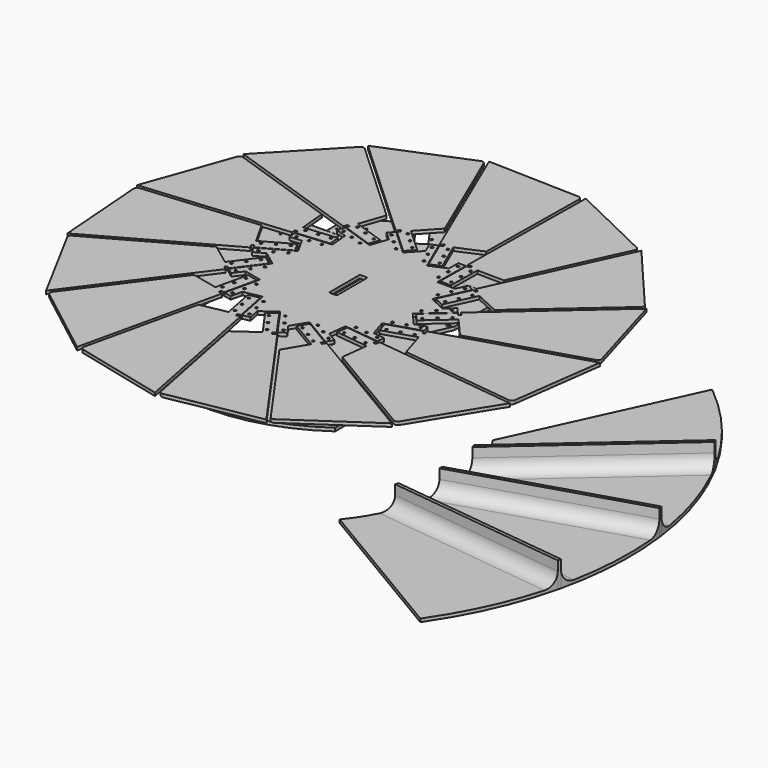
from build123d import *

# Parameters (mm, degrees)
F5_DEPTH = 40
F6_DEPTH = 35
F7_R     = 20
F0_R     = 1.9
F0_R_2   = 1.75
F8_DEPTH = 5
F2_R     = 1.4
F9_DEPTH = 5
F2_R_2   = 1.9
F2_W     = 5
F2_H     = 5
F2_R_3   = 16


with BuildPart() as f5:
    # F4 (on offset) → F5 (new body)
    with BuildSketch(Plane.XY.offset(-180)):
        with BuildLine():
            ThreePointArc((152.4859565585, -92.1641828619), (151.5670252148, -94.5763902457), (150.6219048273, -96.9784574241))
            Line((150.6219048273, -96.9784574241), (430.9555621315, -130.1581322678))
            ThreePointArc((430.9555621315, -130.1581322678), (431.541953989, -127.7107963244), (432.1163824358, -125.2606247814))
            Line((432.1163824358, -125.2606247814), (152.4859565585, -92.1641828619))
        make_face()
        with BuildLine():
            Line((430.9555621315, -130.1581322678), (150.6219048273, -96.9784574241))
            ThreePointArc((150.6219048273, -96.9784574241), (134.6384036274, -129.5048123953), (113.8875354762, -159.217394735))
            Line((113.8875354762, -159.217394735), (354.182792578, -302.1780498209))
            Line((354.182792578, -302.1780498209), (356.7392580084, -297.8810177633))
            ThreePointArc((356.7392580084, -297.8810177634), (401.3722979363, -217.3492897694), (430.9555621315, -130.1581322678))
        make_face()
        with BuildLine():
            ThreePointArc((166.581347197, -30.5797229561), (161.5926160767, -61.8432066107), (152.4859565585, -92.1641828619))
            Line((152.4859565585, -92.1641828619), (432.1163824358, -125.2606247814))
            ThreePointArc((432.1163824358, -125.2606247814), (444.73424073, -35.6541636121), (441.4771291123, 54.7776861707))
            Line((441.4771291123, 54.7776861707), (166.581347197, -30.5797229561))
        make_face()
        with BuildLine():
            ThreePointArc((167.0124499283, -25.2103692451), (166.8121368082, -27.8962695717), (166.581347197, -30.5797229561))
            Line((166.581347197, -30.5797229561), (441.4771291123, 54.7776861707))
            ThreePointArc((441.4771291123, 54.7776861707), (441.1572058027, 57.2949723658), (440.8248859522, 59.8106520411))
            Line((440.8248859522, 59.8106520411), (167.0124499283, -25.2103692451))
        make_face()
        with BuildLine():
            ThreePointArc((162.8378639859, 38.2580484491), (167.0616347314, 6.6643647704), (167.0124499283, -25.2103692451))
            Line((167.0124499283, -25.2103692451), (440.8248859522, 59.8106520411))
            ThreePointArc((440.8248859522, 59.8106520411), (420.64572605, 148.9482124367), (385.0315824556, 233.1167097719))
            Line((385.0315824556, 233.1167097719), (162.8378639859, 38.2580484491))
        make_face()
        with BuildLine():
            ThreePointArc((161.6328579843, 43.8516393894), (162.2522237752, 41.0584766059), (162.8378639859, 38.2580484491))
            Line((162.8378639859, 38.2580484491), (385.0315824556, 233.1167097719))
            ThreePointArc((385.0315824556, 233.1167097719), (383.8207285252, 235.3780934105), (382.598628532, 237.6334192868))
            Line((382.598628532, 237.6334192868), (161.6328579843, 43.8516393894))
        make_face()
        with BuildLine():
            ThreePointArc((129.2130710056, 120.4418545445), (148.8051032395, 83.578368714), (161.6328579843, 43.8516393894))
            Line((161.6328579843, 43.8516393894), (382.598628532, 237.6334192868))
            ThreePointArc((382.598628532, 237.6334192868), (327.625776734, 318.9452816199), (258.2280754908, 388.3541603965))
            Line((258.2280754908, 388.3541603965), (254.2399532921, 391.6461274173))
            Line((254.2399532921, 391.6461274173), (129.2130710056, 120.4418545445))
        make_face()
    extrude(amount=-F5_DEPTH)

    # F4 (on offset) → F6 (cut)
    with BuildSketch(Plane.XY.offset(-180)):
        with BuildLine():
            Line((430.9555621315, -130.1581322678), (150.6219048273, -96.9784574241))
            ThreePointArc((150.6219048273, -96.9784574241), (134.6384036274, -129.5048123953), (113.8875354762, -159.217394735))
            Line((113.8875354762, -159.217394735), (354.182792578, -302.1780498209))
            Line((354.182792578, -302.1780498209), (356.7392580084, -297.8810177633))
            ThreePointArc((356.7392580084, -297.8810177634), (401.3722979363, -217.3492897694), (430.9555621315, -130.1581322678))
        make_face()
        with BuildLine():
            ThreePointArc((166.581347197, -30.5797229561), (161.5926160767, -61.8432066107), (152.4859565585, -92.1641828619))
            Line((152.4859565585, -92.1641828619), (432.1163824358, -125.2606247814))
            ThreePointArc((432.1163824358, -125.2606247814), (444.73424073, -35.6541636121), (441.4771291123, 54.7776861707))
            Line((441.4771291123, 54.7776861707), (166.581347197, -30.5797229561))
        make_face()
        with BuildLine():
            ThreePointArc((162.8378639859, 38.2580484491), (167.0616347314, 6.6643647704), (167.0124499283, -25.2103692451))
            Line((167.0124499283, -25.2103692451), (440.8248859522, 59.8106520411))
            ThreePointArc((440.8248859522, 59.8106520411), (420.64572605, 148.9482124367), (385.0315824556, 233.1167097719))
            Line((385.0315824556, 233.1167097719), (162.8378639859, 38.2580484491))
        make_face()
        with BuildLine():
            ThreePointArc((129.2130710056, 120.4418545445), (148.8051032395, 83.578368714), (161.6328579843, 43.8516393894))
            Line((161.6328579843, 43.8516393894), (382.598628532, 237.6334192868))
            ThreePointArc((382.598628532, 237.6334192868), (327.625776734, 318.9452816199), (258.2280754908, 388.3541603965))
            Line((258.2280754908, 388.3541603965), (254.2399532921, 391.6461274173))
            Line((254.2399532921, 391.6461274173), (129.2130710056, 120.4418545445))
        make_face()
    extrude(amount=-F6_DEPTH, mode=Mode.SUBTRACT)

    # F7
    f7_edges = [f5.edges().sort_by_distance(p)[0] for p in [
        (290.788733, -113.568295, -215),
        (304.029238, 12.098982, -215),
        (273.934723, 135.687379, -215),
        (292.301169, -108.712404, -215),
        (303.918668, 17.300141, -215),
        (272.115743, 140.742529, -215),
    ]]
    fillet(f7_edges, radius=F7_R)


with BuildPart() as f8:
    # F0 (on Top) → F8 (new body)
    with BuildSketch(Plane.XY):
        with BuildLine():
            Line((-99.5654662237, 123.5643549186), (-95.7777457057, 122.2785970574))
            Line((-95.7777457057, 122.2785970574), (-91.9847600151, 133.4523725854))
            Line((-91.9847600151, 133.4523725854), (-78.5983493232, 172.8874668356))
            Line((-78.5983493232, 172.8874668356), (-209.6199457093, 294.0025847368))
            ThreePointArc((-209.6199457093, 294.0025847368), (-213.166642003, 295.3286401438), (-216.6257692473, 293.7885374685))
            Line((-216.6257692473, 293.7885374685), (-315.5944341041, 190.1376257037))
            Line((-315.5944341041, 190.1376257037), (-101.6226788016, 117.5040020898))
            Line((-101.6226788016, 117.5040020898), (-99.5654662237, 123.5643549186))
        make_face()
        Polygon((-96.099185171, 121.3316669279), (-97.5135188184, 117.1651743581), (-49.2200822141, 100.7717616276), (-47.8057485668, 104.9382541974), align=None)
        Polygon((-95.7777457057, 122.2785970574), (-96.099185171, 121.3316669279), (-47.8057485668, 104.9382541974), (-47.4843091015, 105.8851843269), align=None)
        Polygon((-91.9847600151, 133.4523725854), (-95.7777457057, 122.2785970574), (-47.4843091015, 105.8851843269), (-43.6913234109, 117.058959855), align=None)
        with Locations((-69.4452390395, 120.5210155727)):
            Circle(F0_R, mode=Mode.SUBTRACT)
        with Locations((-86.9634464352, 126.4676456808)):
            Circle(F0_R, mode=Mode.SUBTRACT)
        with Locations((-51.9270316439, 114.5743854646)):
            Circle(F0_R_2, mode=Mode.SUBTRACT)
    extrude(amount=F8_DEPTH)


with BuildPart() as f8b:
    # F0 (on Top) → F8, piece 2 (new body)
    with BuildSketch(Plane.XY):
        with BuildLine():
            Line((-141.2157303301, 72.3847316643), (-137.2325106198, 72.750738139))
            Line((-137.2325106198, 72.750738139), (-138.3122297201, 84.5012362844))
            Line((-138.3122297201, 84.5012362844), (-142.122832893, 125.971731256))
            Line((-142.122832893, 125.971731256), (-311.0789736055, 183.324612782))
            ThreePointArc((-311.0789736055, 183.324612782), (-314.858397219, 183.0934533311), (-317.3920510083, 180.2795457245))
            Line((-317.3920510083, 180.2795457245), (-365.6458013342, 45.3355435877))
            Line((-365.6458013342, 45.3355435877), (-140.6301199707, 66.0115801278))
            Line((-140.6301199707, 66.0115801278), (-141.2157303301, 72.3847316643))
        make_face()
        Polygon((-136.7384018791, 67.3733915301), (-85.9523505728, 72.0399740819), (-86.3549576949, 76.4215157632), (-137.1410090012, 71.7549332114), align=None)
        Polygon((-137.1410090012, 71.7549332114), (-86.3549576949, 76.4215157632), (-86.4464593135, 77.4173206908), (-137.2325106198, 72.750738139), align=None)
        Polygon((-137.2325106198, 72.750738139), (-86.4464593135, 77.4173206908), (-87.5261784138, 89.1678188362), (-138.3122297201, 84.5012362844), align=None)
        with Locations((-130.8840871337, 80.1627229771)):
            Circle(F0_R, mode=Mode.SUBTRACT)
        with Locations((-112.4616959736, 81.8555029224)):
            Circle(F0_R, mode=Mode.SUBTRACT)
        with Locations((-94.0393048135, 83.5482828677)):
            Circle(F0_R_2, mode=Mode.SUBTRACT)
    extrude(amount=F8_DEPTH)


with BuildPart() as f8c:
    # F0 (on Top) → F8, piece 3 (new body)
    with BuildSketch(Plane.XY):
        with BuildLine():
            Line((-158.4485117579, 8.6891307106), (-154.9585277296, 10.6436156766))
            Line((-154.9585277296, 10.6436156766), (-160.7242583792, 20.9390685601))
            Line((-160.7242583792, 20.9390685601), (-181.0729875102, 57.2743389249))
            Line((-181.0729875102, 57.2743389249), (-358.7496209015, 40.9481498253))
            ThreePointArc((-358.7496209015, 40.9481498253), (-362.1082751571, 39.1997450856), (-363.2783637337, 35.5985827364))
            Line((-363.2783637337, 35.5985827364), (-352.4736877258, -107.3054658752))
            Line((-352.4736877258, -107.3054658752), (-155.3213358123, 3.1051562654))
            Line((-155.3213358123, 3.1051562654), (-158.4485117579, 8.6891307106))
        make_face()
        Polygon((-152.3199730255, 5.9321372384), (-107.8226766648, 30.8518205548), (-109.9726101274, 34.6908029859), (-154.4699064881, 9.7711196695), align=None)
        Polygon((-154.4699064881, 9.7711196695), (-109.9726101274, 34.6908029859), (-110.4612313689, 35.563298993), (-154.9585277296, 10.6436156766), align=None)
        Polygon((-154.9585277296, 10.6436156766), (-110.4612313689, 35.563298993), (-116.2269620185, 45.8587518764), (-160.7242583792, 20.9390685601), align=None)
        with Locations((-152.1736801223, 19.9969372152)):
            Circle(F0_R, mode=Mode.SUBTRACT)
        with Locations((-136.0325039914, 29.0364301829)):
            Circle(F0_R, mode=Mode.SUBTRACT)
        with Locations((-119.8913278606, 38.0759231506)):
            Circle(F0_R_2, mode=Mode.SUBTRACT)
    extrude(amount=F8_DEPTH)


with BuildPart() as f8d:
    # F0 (on Top) → F8, piece 4 (new body)
    with BuildSketch(Plane.XY):
        with BuildLine():
            Line((-148.2841060431, -56.5088998812), (-145.8908076408, -53.3038846304))
            Line((-145.8908076408, -53.3038846304), (-155.3456026306, -46.2436543437))
            Line((-155.3456026306, -46.2436543437), (-188.7139775905, -21.3263069273))
            Line((-188.7139775905, -21.3263069273), (-344.3891996057, -108.5086202385))
            ThreePointArc((-344.3891996057, -108.5086202385), (-346.7463426701, -111.4719552037), (-346.3505470892, -115.2376986098))
            Line((-346.3505470892, -115.2376986098), (-278.3556713867, -241.3923854486))
            Line((-278.3556713867, -241.3923854486), (-143.1560816419, -60.3381773248))
            Line((-143.1560816419, -60.3381773248), (-148.2841060431, -56.5088998812))
        make_face()
        Polygon((-141.5640370523, -56.5348374735), (-111.0494824232, -15.6708930263), (-114.574999199, -13.0382647838), (-145.0895538282, -53.902209231), align=None)
        Polygon((-145.0895538282, -53.902209231), (-114.574999199, -13.0382647838), (-115.3762530117, -12.4399401832), (-145.8908076408, -53.3038846304), align=None)
        Polygon((-145.8908076408, -53.3038846304), (-115.3762530117, -12.4399401832), (-124.8310480015, -5.3797098964), (-155.3456026306, -46.2436543437), align=None)
        with Locations((-147.1510613631, -43.6265006577)):
            Circle(F0_R, mode=Mode.SUBTRACT)
        with Locations((-136.0820562526, -28.8033051229)):
            Circle(F0_R, mode=Mode.SUBTRACT)
        with Locations((-125.013051142, -13.9801095881)):
            Circle(F0_R_2, mode=Mode.SUBTRACT)
    extrude(amount=F8_DEPTH)


with BuildPart() as f8e:
    # F0 (on Top) → F8, piece 5 (new body)
    with BuildSketch(Plane.XY):
        with BuildLine():
            Line((-112.4800312747, -111.9360283163), (-111.5972415346, -108.0346590343))
            Line((-111.5972415346, -108.0346590343), (-123.1062809166, -105.430429301))
            Line((-123.1062809166, -105.430429301), (-163.7246065327, -96.2394405683))
            Line((-163.7246065327, -96.2394405683), (-270.4807570204, -239.2032640931))
            ThreePointArc((-270.4807570204, -239.2032640931), (-271.4288174439, -242.8691417473), (-269.5355743571, -246.1483349647))
            Line((-269.5355743571, -246.1483349647), (-156.107430683, -333.740368597))
            Line((-156.107430683, -333.740368597), (-106.2378404235, -113.3484919005))
            Line((-106.2378404235, -113.3484919005), (-112.4800312747, -111.9360283163))
        make_face()
        Polygon((-106.3303930039, -109.2264251834), (-95.0748238178, -59.4839668375), (-99.366330028, -58.5128981234), (-110.6218992141, -108.2553564693), align=None)
        Polygon((-110.6218992141, -108.2553564693), (-99.366330028, -58.5128981234), (-100.3416723485, -58.2922006884), (-111.5972415346, -108.0346590343), align=None)
        Polygon((-111.5972415346, -108.0346590343), (-100.3416723485, -58.2922006884), (-111.8507117305, -55.6879709551), (-123.1062809166, -105.430429301), align=None)
        with Locations((-116.6846872689, -99.7065202326)):
            Circle(F0_R, mode=Mode.SUBTRACT)
        with Locations((-112.601784721, -81.6626873032)):
            Circle(F0_R, mode=Mode.SUBTRACT)
        with Locations((-108.5188821731, -63.6188543738)):
            Circle(F0_R_2, mode=Mode.SUBTRACT)
    extrude(amount=F8_DEPTH)


with BuildPart() as f8f:
    # F0 (on Top) → F8, piece 6 (new body)
    with BuildSketch(Plane.XY):
        with BuildLine():
            Line((-57.2271372499, -148.0084005487), (-58.007498538, -144.085259427))
            Line((-58.007498538, -144.085259427), (-69.5807648467, -146.3873252268))
            Line((-69.5807648467, -146.3873252268), (-110.425763614, -154.5119006273))
            Line((-110.425763614, -154.5119006273), (-149.8037343057, -328.5374904926))
            ThreePointArc((-149.8037343057, -328.5374904926), (-149.1787838281, -332.272047286), (-146.1154521648, -334.4976880168))
            Line((-146.1154521648, -334.4976880168), (-6.8667970226, -368.381610079))
            Line((-6.8667970226, -368.381610079), (-50.9501114553, -146.7598224878))
            Line((-50.9501114553, -146.7598224878), (-57.2271372499, -148.0084005487))
        make_face()
        Polygon((-52.7112580238, -143.0317716882), (-62.6608644466, -93.0117223876), (-66.9763196804, -93.8701198045), (-57.0267132576, -143.890169105), align=None)
        Polygon((-57.0267132576, -143.890169105), (-66.9763196804, -93.8701198045), (-67.9571049608, -94.0652101265), (-58.007498538, -144.085259427), align=None)
        Polygon((-58.007498538, -144.085259427), (-67.9571049608, -94.0652101265), (-79.5303712695, -96.3672759263), (-69.5807648467, -146.3873252268), align=None)
        with Locations((-69.6516416561, -120.4018489665)):
            Circle(F0_R, mode=Mode.SUBTRACT)
        with Locations((-66.0424706988, -138.5463766539)):
            Circle(F0_R, mode=Mode.SUBTRACT)
        with Locations((-73.2608126134, -102.257321279)):
            Circle(F0_R_2, mode=Mode.SUBTRACT)
    extrude(amount=F8_DEPTH)


with BuildPart() as f8g:
    # F0 (on Top) → F8, piece 7 (new body)
    with BuildSketch(Plane.XY):
        with BuildLine():
            Line((7.9208486977, -158.488775712), (5.6122679375, -155.2222094914))
            Line((5.6122679375, -155.2222094914), (-4.0241024134, -162.0325227338))
            Line((-4.0241024134, -162.0325227338), (-38.0333029799, -186.0678493712))
            Line((-38.0333029799, -186.0678493712), (-3.2242850054, -361.0646001165))
            ThreePointArc((-3.2242850054, -361.0646001165), (-1.1343832418, -364.2220972521), (2.569359124, -365.0093519947))
            Line((2.569359124, -365.0093519947), (143.5611682258, -339.3263245364))
            Line((143.5611682258, -339.3263245364), (13.1473546507, -154.7950464958))
            Line((13.1473546507, -154.7950464958), (7.9208486977, -158.488775712))
        make_face()
        Polygon((10.0221323354, -152.1056254652), (-19.4122723565, -110.4569061519), (-23.0054951992, -112.9963449881), (6.4289094927, -154.6450643014), align=None)
        Polygon((6.4289094927, -154.6450643014), (-23.0054951992, -112.9963449881), (-23.8221367544, -113.5734901781), (5.6122679375, -155.2222094914), align=None)
        Polygon((5.6122679375, -155.2222094914), (-23.8221367544, -113.5734901781), (-33.4585071053, -120.3838034206), (-4.0241024134, -162.0325227338), align=None)
        with Locations((-3.9809109679, -153.4303058975)):
            Circle(F0_R, mode=Mode.SUBTRACT)
        with Locations((-25.3352829992, -123.2145683565)):
            Circle(F0_R_2, mode=Mode.SUBTRACT)
        with Locations((-14.6580969835, -138.322437127)):
            Circle(F0_R, mode=Mode.SUBTRACT)
    extrude(amount=F8_DEPTH)


with BuildPart() as f8h:
    # F0 (on Top) → F8, piece 8 (new body)
    with BuildSketch(Plane.XY):
        with BuildLine():
            Line((71.6992479467, -141.5650017295), (68.2616223007, -139.5198293852))
            Line((68.2616223007, -139.5198293852), (62.228363885, -149.6608250409))
            Line((62.228363885, -149.6608250409), (40.9354612612, -185.4509765855))
            Line((40.9354612612, -185.4509765855), (143.9126724641, -331.1603602114))
            ThreePointArc((143.9126724641, -331.1603602114), (147.1061625126, -333.1948377495), (150.8099048784, -332.4075830069))
            Line((150.8099048784, -332.4075830069), (269.1661032757, -251.5984347986))
            Line((269.1661032757, -251.5984347986), (74.9715236976, -136.0648006959))
            Line((74.9715236976, -136.0648006959), (71.6992479467, -141.5650017295))
        make_face()
        Polygon((71.0226049655, -134.8790347631), (27.192877979, -108.8030873731), (24.9431884002, -112.5844755837), (68.7729153868, -138.6604229737), align=None)
        Polygon((68.7729153868, -138.6604229737), (24.9431884002, -112.5844755837), (24.4318953141, -113.4438819952), (68.2616223007, -139.5198293852), align=None)
        Polygon((68.2616223007, -139.5198293852), (24.4318953141, -113.4438819952), (18.3986368984, -123.584877651), (62.228363885, -149.6608250409), align=None)
        with Locations((58.7689844349, -141.7847413808)):
            Circle(F0_R, mode=Mode.SUBTRACT)
        with Locations((42.8699658221, -132.3258192884)):
            Circle(F0_R, mode=Mode.SUBTRACT)
        with Locations((26.9709472093, -122.866897196)):
            Circle(F0_R_2, mode=Mode.SUBTRACT)
    extrude(amount=F8_DEPTH)


with BuildPart() as f8i:
    # F0 (on Top) → F8, piece 9 (new body)
    with BuildSketch(Plane.XY):
        with BuildLine():
            Line((123.0801958586, -100.1633528702), (119.1079220308, -99.6932032804))
            Line((119.1079220308, -99.6932032804), (117.7209807408, -111.4114110725))
            Line((117.7209807408, -111.4114110725), (112.8261123632, -152.7679451789))
            Line((112.8261123632, -152.7679451789), (266.165821459, -243.9954855283))
            ThreePointArc((266.165821459, -243.9954855283), (269.910716351, -244.5551638199), (272.9740480143, -242.329523089))
            Line((272.9740480143, -242.329523089), (348.229773772, -120.3668899841))
            Line((348.229773772, -120.3668899841), (123.8324352023, -93.8077147457))
            Line((123.8324352023, -93.8077147457), (123.0801958586, -100.1633528702))
        make_face()
        Polygon((119.2254594282, -98.7001348234), (119.742623977, -94.3306336128), (69.0961326723, -88.3362263425), (68.5789681235, -92.7057275531), align=None)
        Polygon((119.1079220308, -99.6932032804), (119.2254594282, -98.7001348234), (68.5789681235, -92.7057275531), (68.4614307261, -93.69879601), align=None)
        Polygon((117.7209807408, -111.4114110725), (119.1079220308, -99.6932032804), (68.4614307261, -93.69879601), (67.0744894361, -105.4170038021), align=None)
        with Locations((74.613655622, -101.2744232995)):
            Circle(F0_R_2, mode=Mode.SUBTRACT)
        with Locations((92.9854220757, -103.4488651525)):
            Circle(F0_R, mode=Mode.SUBTRACT)
        with Locations((111.3571885294, -105.6233070055)):
            Circle(F0_R, mode=Mode.SUBTRACT)
    extrude(amount=F8_DEPTH)


with BuildPart() as f8j:
    # F0 (on Top) → F8, piece 10 (new body)
    with BuildSketch(Plane.XY):
        with BuildLine():
            Line((153.179459758, -41.4425503442), (149.3593799802, -42.6287166441))
            Line((149.3593799802, -42.6287166441), (152.8585705649, -53.8979519887))
            Line((152.8585705649, -53.8979519887), (165.2081036445, -93.6699481977))
            Line((165.2081036445, -93.6699481977), (342.396481883, -114.6415747679))
            ThreePointArc((342.396481883, -114.6415747679), (346.0452552704, -113.6296803519), (347.9384983572, -110.3504871345))
            Line((347.9384983572, -110.3504871345), (367.0813528149, 31.6771836076))
            Line((367.0813528149, 31.6771836076), (151.2815936782, -35.3304226997))
            Line((151.2815936782, -35.3304226997), (153.179459758, -41.4425503442))
        make_face()
        Polygon((149.0628384052, -41.6736966997), (147.7580554753, -37.471608944), (99.052038308, -52.5952292678), (100.3568212379, -56.7973170234), align=None)
        Polygon((149.3593799802, -42.6287166441), (149.0628384052, -41.6736966997), (100.3568212379, -56.7973170234), (100.6533628129, -57.7523369679), align=None)
        Polygon((152.8585705649, -53.8979519887), (149.3593799802, -42.6287166441), (100.6533628129, -57.7523369679), (104.1525533976, -69.0215723125), align=None)
        with Locations((109.3549851339, -62.1706815653)):
            Circle(F0_R_2, mode=Mode.SUBTRACT)
        with Locations((127.0228541064, -56.6846624283)):
            Circle(F0_R, mode=Mode.SUBTRACT)
        with Locations((144.6907230788, -51.1986432912)):
            Circle(F0_R, mode=Mode.SUBTRACT)
    extrude(amount=F8_DEPTH)


with BuildPart() as f8k:
    # F0 (on Top) → F8, piece 11 (new body)
    with BuildSketch(Plane.XY):
        with BuildLine():
            Line((156.7926034736, 24.4440456301), (153.7852442437, 21.8066623697))
            Line((153.7852442437, 21.8066623697), (161.5655248619, 12.9349526414))
            Line((161.5655248619, 12.9349526414), (189.0241129372, -18.3755662084))
            Line((189.0241129372, -18.3755662084), (359.423680015, 34.5349057558))
            ThreePointArc((359.423680015, 34.5349057558), (362.3454258312, 36.9434071422), (362.7412214121, 40.7091505482))
            Line((362.7412214121, 40.7091505482), (322.4612311267, 178.2439843753))
            Line((322.4612311267, 178.2439843753), (152.5727902569, 29.2558203979))
            Line((152.5727902569, 29.2558203979), (156.7926034736, 24.4440456301))
        make_face()
        Polygon((153.1258984286, 22.5585021771), (150.2247768421, 25.8665973301), (111.8809466607, -7.7600392401), (114.7820682471, -11.068134393), align=None)
        Polygon((153.7852442437, 21.8066623697), (153.1258984286, 22.5585021771), (114.7820682471, -11.068134393), (115.4414140622, -11.8199742004), align=None)
        Polygon((161.5655248619, 12.9349526414), (153.7852442437, 21.8066623697), (115.4414140622, -11.8199742004), (123.2216946804, -20.6916839287), align=None)
        with Locations((125.1878442573, -12.3170641856)):
            Circle(F0_R_2, mode=Mode.SUBTRACT)
        with Locations((139.0968806956, -0.1191666062)):
            Circle(F0_R, mode=Mode.SUBTRACT)
        with Locations((153.005917134, 12.0787309731)):
            Circle(F0_R, mode=Mode.SUBTRACT)
    extrude(amount=F8_DEPTH)


with BuildPart() as f8l:
    # F0 (on Top) → F8, piece 12 (new body)
    with BuildSketch(Plane.XY):
        with BuildLine():
            Line((133.2948816325, 86.1040440477), (131.6202426823, 82.4714713524))
            Line((131.6202426823, 82.4714713524), (142.3363321335, 77.5312864495))
            Line((142.3363321335, 77.5312864495), (180.1561358729, 60.0961181152))
            Line((180.1561358729, 60.0961181152), (314.3032586109, 177.7399873346))
            ThreePointArc((314.3032586109, 177.7399873346), (315.9927804609, 181.128643921), (314.8226918843, 184.7298062702))
            Line((314.8226918843, 184.7298062702), (222.0846331084, 293.9907809487))
            Line((222.0846331084, 293.9907809487), (127.48276532, 88.783466368))
            Line((127.48276532, 88.783466368), (133.2948816325, 86.1040440477))
        make_face()
        Polygon((130.7120995085, 82.89013109), (126.7162695437, 84.7322339351), (105.3646229293, 38.41693207), (109.3604528941, 36.5748292249), align=None)
        Polygon((131.6202426823, 82.4714713524), (130.7120995085, 82.89013109), (109.3604528941, 36.5748292249), (110.2685960679, 36.1561694873), align=None)
        Polygon((142.3363321335, 77.5312864495), (131.6202426823, 82.4714713524), (110.2685960679, 36.1561694873), (120.9846855191, 31.2159845844), align=None)
        with Locations((119.3745878127, 39.6662854889)):
            Circle(F0_R_2, mode=Mode.SUBTRACT)
        with Locations((127.1197929571, 56.4669342046)):
            Circle(F0_R, mode=Mode.SUBTRACT)
        with Locations((134.8649981016, 73.2675829204)):
            Circle(F0_R, mode=Mode.SUBTRACT)
    extrude(amount=F8_DEPTH)


with BuildPart() as f8m:
    # F0 (on Top) → F8, piece 13 (new body)
    with BuildSketch(Plane.XY):
        with BuildLine():
            Line((86.7492638111, 132.8758710188), (86.6969054289, 128.8762137085))
            Line((86.6969054289, 128.8762137085), (98.4958944942, 128.7217564808))
            Line((98.4958944942, 128.7217564808), (140.1375262491, 128.1766376605))
            Line((140.1375262491, 128.1766376605), (214.8369484374, 290.2122103861))
            ThreePointArc((214.8369484374, 290.2122103861), (215.0021126446, 293.9950926638), (212.4684588553, 296.8090002704))
            Line((212.4684588553, 296.8090002704), (83.3075844501, 358.9039006737))
            Line((83.3075844501, 358.9039006737), (80.3498121147, 132.9596444305))
            Line((80.3498121147, 132.9596444305), (86.7492638111, 132.8758710188))
        make_face()
        Polygon((85.6969911013, 128.8893033041), (81.29736806, 128.9468975246), (80.6297986858, 77.9512668184), (85.0294217272, 77.8936725978), align=None)
        Polygon((86.6969054289, 128.8762137085), (85.6969911013, 128.8893033041), (85.0294217272, 77.8936725978), (86.0293360547, 77.8805830023), align=None)
        Polygon((98.4958944942, 128.7217564808), (86.6969054289, 128.8762137085), (86.0293360547, 77.8805830023), (97.8283251201, 77.7261257745), align=None)
        with Locations((92.9203806512, 84.7909740454)):
            Circle(F0_R_2, mode=Mode.SUBTRACT)
        with Locations((93.1625381693, 103.2893891055)):
            Circle(F0_R, mode=Mode.SUBTRACT)
        with Locations((93.4046956874, 121.7878041656)):
            Circle(F0_R, mode=Mode.SUBTRACT)
    extrude(amount=F8_DEPTH)


with BuildPart() as f8n:
    # F0 (on Top) → F8, piece 14 (new body)
    with BuildSketch(Plane.XY):
        with BuildLine():
            Line((25.2039101845, 156.6722527514), (26.7828856101, 152.9970879108))
            Line((26.7828856101, 152.9970879108), (37.6246218898, 157.6550654161))
            Line((37.6246218898, 157.6550654161), (75.8878652273, 174.0942521062))
            Line((75.8878652273, 174.0942521062), (78.2233781467, 352.5041057668))
            ThreePointArc((78.2233781467, 352.5041057668), (76.8356263192, 356.0271190235), (73.3764990749, 357.5672216988))
            Line((73.3764990749, 357.5672216988), (-69.8741023853, 361.7592754327))
            Line((-69.8741023853, 361.7592754327), (19.3236464396, 154.1458920705))
            Line((19.3236464396, 154.1458920705), (25.2039101845, 156.6722527514))
        make_face()
        Polygon((25.8640943999, 152.6023440544), (21.8214130753, 150.8654710863), (41.9533497509, 104.0071193687), (45.9960310755, 105.7439923368), align=None)
        Polygon((26.7828856101, 152.9970879108), (25.8640943999, 152.6023440544), (45.9960310755, 105.7439923368), (46.9148222857, 106.1387361932), align=None)
        Polygon((37.6246218898, 157.6550654161), (26.7828856101, 152.9970879108), (46.9148222857, 106.1387361932), (57.7565585654, 110.7967136986), align=None)
        with Locations((43.0966341769, 132.2521702754)):
            Circle(F0_R, mode=Mode.SUBTRACT)
        with Locations((50.39939552, 115.2545328877)):
            Circle(F0_R_2, mode=Mode.SUBTRACT)
        with Locations((35.7938728338, 149.2498076632)):
            Circle(F0_R, mode=Mode.SUBTRACT)
    extrude(amount=F8_DEPTH)


with BuildPart() as f8o:
    # F0 (on Top) → F8, piece 15 (new body)
    with BuildSketch(Plane.XY):
        with BuildLine():
            Line((-40.6994284833, 153.3785786605), (-37.7621384456, 150.6633756784))
            Line((-37.7621384456, 150.6633756784), (-29.7522896483, 159.3283812897))
            Line((-29.7522896483, 159.3283812897), (-1.4834971118, 189.909388766))
            Line((-1.4834971118, 189.9093887661), (-71.9157248626, 353.844838861))
            ThreePointArc((-71.9157248626, 353.844838861), (-74.6164378265, 356.4988220992), (-78.402924, 356.4988220992))
            Line((-78.402924, 356.4988220992), (-210.9739221319, 302.0631849895))
            Line((-210.9739221319, 302.0631849895), (-45.0437532547, 148.6789146001))
            Line((-45.0437532547, 148.6789146001), (-40.6994284833, 153.3785786605))
        make_face()
        Polygon((-38.4409391911, 149.929053169), (-41.4276624714, 146.6980341274), (-3.9772144902, 112.0791961053), (-0.9904912099, 115.3102151468), align=None)
        Polygon((-37.7621384456, 150.6633756784), (-38.4409391911, 149.929053169), (-0.9904912099, 115.3102151468), (-0.3116904643, 116.0445376562), align=None)
        Polygon((-29.7522896483, 159.3283812897), (-37.7621384456, 150.6633756784), (-0.3116904643, 116.0445376562), (7.6981583329, 124.7095432676), align=None)
        with Locations((-0.8361029608, 125.7895359391)):
            Circle(F0_R_2, mode=Mode.SUBTRACT)
        with Locations((-28.0060358099, 150.9051635238)):
            Circle(F0_R, mode=Mode.SUBTRACT)
        with Locations((-14.4210693853, 138.3473497315)):
            Circle(F0_R, mode=Mode.SUBTRACT)
    extrude(amount=F8_DEPTH)


with BuildPart() as f8p:
    # F0 (on Top) → F8, piece 16 (new body)
    with BuildSketch(Plane.XY):
        Polygon((-49.5415216794, 99.8248314982), (-97.8349582837, 116.2182442286), (-101.6279439742, 105.0444687006), (-84.4318141394, 99.2071691922), (-53.33450737, 88.6510559701), align=None)
        with Locations((-93.3922357413, 107.5290430909)):
            Circle(F0_R, mode=Mode.SUBTRACT)
        with Locations((-75.8740283456, 101.5824129828)):
            Circle(F0_R, mode=Mode.SUBTRACT)
        with Locations((-58.3558209499, 95.6357828747)):
            Circle(F0_R, mode=Mode.SUBTRACT)
        Polygon((-84.7811298539, 59.2936710089), (-85.8608489541, 71.0441691543), (-136.6469002604, 66.3775866025), (-135.5671811602, 54.6270884571), (-117.4834912539, 56.2887461292), align=None)
        with Locations((-129.0540547605, 60.2466244256)):
            Circle(F0_R, mode=Mode.SUBTRACT)
        with Locations((-110.6316636003, 61.9394043709)):
            Circle(F0_R, mode=Mode.SUBTRACT)
        with Locations((-92.2092724402, 63.6321843162)):
            Circle(F0_R, mode=Mode.SUBTRACT)
        Polygon((-101.5683247736, 19.6838716642), (-107.3340554233, 29.9793245477), (-151.831351784, 5.0596412314), (-146.0656211343, -5.2358116521), (-130.2212054265, 3.6374874933), align=None)
        with Locations((-142.4012552923, 2.5470170737)):
            Circle(F0_R, mode=Mode.SUBTRACT)
        with Locations((-126.2600791615, 11.5865100414)):
            Circle(F0_R, mode=Mode.SUBTRACT)
        with Locations((-110.1189030306, 20.6260030091)):
            Circle(F0_R, mode=Mode.SUBTRACT)
        Polygon((-100.7934336208, -23.3294479136), (-110.2482286105, -16.2692176268), (-140.7627832396, -57.1331620741), (-131.3079882499, -64.1933923608), (-120.4424901584, -49.6427257757), align=None)
        with Locations((-131.1259851093, -55.5929926691)):
            Circle(F0_R, mode=Mode.SUBTRACT)
        with Locations((-120.0569799988, -40.7697971343)):
            Circle(F0_R, mode=Mode.SUBTRACT)
        with Locations((-108.9879748882, -25.9466015996)):
            Circle(F0_R, mode=Mode.SUBTRACT)
        Polygon((-82.5904421153, -62.3088940057), (-94.0994814973, -59.7046642725), (-105.3550506834, -109.4471226184), (-93.8460113014, -112.0513523517), (-89.8381741562, -94.3392607681), align=None)
        with Locations((-97.1778408588, -104.120468933)):
            Circle(F0_R, mode=Mode.SUBTRACT)
        with Locations((-93.0949383109, -86.0766360036)):
            Circle(F0_R, mode=Mode.SUBTRACT)
        with Locations((-89.012035763, -68.0328030742)):
            Circle(F0_R, mode=Mode.SUBTRACT)
        Polygon((-50.1068128574, -90.5145662658), (-61.6800791662, -92.8166320656), (-51.7304727434, -142.8366813661), (-40.1572064346, -140.5346155664), (-43.7000216883, -122.7236805284), align=None)
        with Locations((-46.4267650907, -134.6445702136)):
            Circle(F0_R, mode=Mode.SUBTRACT)
        with Locations((-50.035936048, -116.5000425262)):
            Circle(F0_R, mode=Mode.SUBTRACT)
        with Locations((-53.6451070053, -98.3555148387)):
            Circle(F0_R, mode=Mode.SUBTRACT)
        Polygon((-8.9592604505, -103.0694477195), (-18.5956308014, -109.8797609619), (10.8387738905, -151.5284802752), (20.4751442414, -144.7181670327), (9.9942615319, -129.8880610158), align=None)
        with Locations((-9.002451896, -111.6716645558)):
            Circle(F0_R, mode=Mode.SUBTRACT)
        with Locations((12.3519201354, -141.8874020968)):
            Circle(F0_R, mode=Mode.SUBTRACT)
        with Locations((1.6747341197, -126.7795333263)):
            Circle(F0_R, mode=Mode.SUBTRACT)
        Polygon((33.7374294807, -97.8026853059), (27.704171065, -107.9436809616), (71.5338980516, -134.0196283516), (77.5671564673, -123.8786326958), (61.9604461381, -114.5936157575), align=None)
        with Locations((37.1968089309, -105.678768966)):
            Circle(F0_R, mode=Mode.SUBTRACT)
        with Locations((68.9948461564, -124.5966131508)):
            Circle(F0_R, mode=Mode.SUBTRACT)
        with Locations((53.0958275436, -115.1376910584)):
            Circle(F0_R, mode=Mode.SUBTRACT)
        Polygon((121.2471026645, -81.6193573638), (103.2131067141, -79.4848932844), (70.6006113598, -75.6249500935), (69.2136700698, -87.3431578855), (119.8601613745, -93.3375651559), align=None)
        with Locations((76.9644035712, -81.4130541604)):
            Circle(F0_R, mode=Mode.SUBTRACT)
        with Locations((95.3361700249, -83.5874960134)):
            Circle(F0_R, mode=Mode.SUBTRACT)
        with Locations((113.7079364785, -85.7619378664)):
            Circle(F0_R, mode=Mode.SUBTRACT)
        Polygon((143.9623233156, -25.247353655), (126.6192834776, -30.6325106648), (95.2563061483, -40.3709739787), (98.755496733, -51.6402093233), (147.4615139003, -36.5165889996), align=None)
        with Locations((103.4241536344, -43.0702826762)):
            Circle(F0_R, mode=Mode.SUBTRACT)
        with Locations((121.0920226069, -37.5842635392)):
            Circle(F0_R, mode=Mode.SUBTRACT)
        with Locations((138.7598915793, -32.0982444021)):
            Circle(F0_R, mode=Mode.SUBTRACT)
        Polygon((141.7851504089, 35.4901468658), (128.1318358277, 23.5165113363), (103.4413202274, 1.8635102957), (111.2216008456, -7.0081994326), (149.565431027, 26.6184371375), align=None)
        with Locations((112.0009279553, 2.719731964)):
            Circle(F0_R, mode=Mode.SUBTRACT)
        with Locations((125.9099643936, 14.9176295433)):
            Circle(F0_R, mode=Mode.SUBTRACT)
        with Locations((139.819000832, 27.1155271227)):
            Circle(F0_R, mode=Mode.SUBTRACT)
        Polygon((115.0920369187, 90.0910785756), (107.489229722, 73.5993148865), (93.7403903043, 43.7757767105), (104.4564797555, 38.8355918076), (125.8081263699, 85.1508936727), align=None)
        with Locations((101.2117243362, 48.0394802396)):
            Circle(F0_R, mode=Mode.SUBTRACT)
        with Locations((108.9569294806, 64.8401289554)):
            Circle(F0_R, mode=Mode.SUBTRACT)
        with Locations((116.7021346251, 81.6407776711)):
            Circle(F0_R, mode=Mode.SUBTRACT)
        Polygon((68.498464667, 129.1144443479), (68.2607592884, 110.9561282641), (67.8308952929, 78.1188136417), (79.6298843583, 77.9643564139), (80.2974537324, 128.9599871202), align=None)
        with Locations((72.9220940997, 85.0527659568)):
            Circle(F0_R, mode=Mode.SUBTRACT)
        with Locations((73.1642516178, 103.5511810169)):
            Circle(F0_R, mode=Mode.SUBTRACT)
        with Locations((73.4064091359, 122.0495960771)):
            Circle(F0_R, mode=Mode.SUBTRACT)
        Polygon((10.0608855854, 145.8127497246), (17.2293834443, 129.1276190601), (30.192822261, 98.954398007), (41.0345585407, 103.6123755124), (20.9026218651, 150.47072723), align=None)
        with Locations((32.023571317, 107.35965576)):
            Circle(F0_R, mode=Mode.SUBTRACT)
        with Locations((24.7208099739, 124.3572931477)):
            Circle(F0_R, mode=Mode.SUBTRACT)
        with Locations((17.4180486308, 141.3549305355)):
            Circle(F0_R, mode=Mode.SUBTRACT)
        Polygon((-50.1163120143, 137.2987060067), (-36.7811093213, 124.971771433), (-12.665864033, 102.6798679845), (-4.6560152358, 111.3448735958), (-42.106463217, 145.963711618), align=None)
        with Locations((-27.997084296, 123.6608995428)):
            Circle(F0_R, mode=Mode.SUBTRACT)
        with Locations((-14.4121178714, 111.1030857504)):
            Circle(F0_R, mode=Mode.SUBTRACT)
        with Locations((-41.5820507206, 136.2187133351)):
            Circle(F0_R, mode=Mode.SUBTRACT)
        Polygon((-45.7538011614, 98.5390736369), (-49.5415216794, 99.8248314982), (-53.33450737, 88.6510559701), (-84.4318141394, 99.2071691922), (-81.8776292438, 71.410175629), (-85.8608489541, 71.0441691543), (-84.7811298539, 59.2936710089), (-117.4834912539, 56.2887461292), (-103.844071395, 31.9338095137), (-107.3340554233, 29.9793245477), (-101.5683247736, 19.6838716642), (-130.2212054265, 3.6374874933), (-107.8549302082, -13.0642023761), (-110.2482286105, -16.2692176268), (-100.7934336208, -23.3294479136), (-120.4424901584, -49.6427257757), (-93.2166917572, -55.8032949905), (-94.0994814973, -59.7046642725), (-82.5904421153, -62.3088940057), (-89.8381741562, -94.3392607681), (-62.4604404543, -88.893490944), (-61.6800791662, -92.8166320656), (-50.1068128574, -90.5145662658), (-43.7000216883, -122.7236805284), (-20.9042115615, -106.6131947413), (-18.5956308014, -109.8797609619), (-8.9592604505, -103.0694477195), (9.9942615319, -129.8880610158), (24.266545419, -105.8985086173), (27.704171065, -107.9436809616), (33.7374294807, -97.8026853059), (61.9604461381, -114.5936157575), (65.241396242, -86.8730082957), (69.2136700698, -87.3431578855), (70.6006113598, -75.6249500935), (103.2131067141, -79.4848932844), (94.9354169552, -52.8263756232), (98.755496733, -51.6402093233), (95.2563061483, -40.3709739787), (126.6192834776, -30.6325106648), (108.2142416157, -9.645582693), (111.2216008456, -7.0081994326), (103.4413202274, 1.8635102957), (128.1318358277, 23.5165113363), (102.7818408053, 35.2030191123), (104.4564797555, 38.8355918076), (93.7403903043, 43.7757767105), (107.489229722, 73.5993148865), (79.577525976, 73.9646991036), (79.6298843583, 77.9643564139), (67.8308952929, 78.1188136417), (68.2607592884, 110.9561282641), (42.6135339663, 99.9372106718), (41.0345585407, 103.6123755124), (30.192822261, 98.954398007), (17.2293834443, 129.1276190601), (-1.718725198, 108.6296706137), (-4.6560152358, 111.3448735958), (-12.665864033, 102.6798679845), (-36.7811093213, 124.971771433), align=None)
        with BuildLine():
            ThreePointArc((6.05, -28.05), (5.4642135624, -29.4642135624), (4.05, -30.05))
            Line((4.05, -30.05), (-4.05, -30.05))
            ThreePointArc((-4.05, -30.05), (-5.4642135624, -29.4642135624), (-6.05, -28.05))
            Line((-6.05, -28.05), (-6.05, 28.05))
            ThreePointArc((-6.05, 28.05), (-5.4642135624, 29.4642135624), (-4.05, 30.05))
            Line((-4.05, 30.05), (4.05, 30.05))
            ThreePointArc((4.05, 30.05), (5.4642135624, 29.4642135624), (6.05, 28.05))
            Line((6.05, 28.05), (6.05, -28.05))
        make_face(mode=Mode.SUBTRACT)
    extrude(amount=F8_DEPTH)


with BuildPart() as f9:
    # F2 (on offset) → F9 (new body)
    with BuildSketch(Plane.XY.offset(-53)):
        with BuildLine():
            Line((158.9568503056, -191.0250148557), (90, -150))
            Line((90, -150), (77.2426406871, -150))
            ThreePointArc((77.2426406871, -150), (74.4710020896, -151.8519497029), (75.1213203436, -155.1213203436))
            Line((75.1213203436, -155.1213203436), (90, -170))
            Line((90, -170), (-61.777287397, -170))
            Line((-61.777287397, -170), (-41.777287397, -150))
            Line((-41.777287397, -150), (-174, -150))
            Line((-174, -150), (-174, -165))
            Line((-174, -165), (-154, -157.7205953147))
            Line((-154, -157.7205953147), (-154, -175))
            Line((-154, -175), (-174, -175))
            Line((-174, -175), (-174, -212.953046468))
            ThreePointArc((-174, -212.953046468), (-9.453167429, -274.8374749294), (158.9568503056, -224.4052578281))
            Line((158.9568503056, -224.4052578281), (158.9568503056, -191.0250148557))
        make_face()
        with Locations((-141.594180879, -206.8316656304)):
            Circle(F2_R, mode=Mode.SUBTRACT)
        with Locations((-168.0623851696, -185.9658158301)):
            Circle(F2_R, mode=Mode.SUBTRACT)
        with Locations((-79.0985290331, -237.8480032942)):
            Circle(F2_R, mode=Mode.SUBTRACT)
        with Locations((-110.2928076438, -225.0860869718)):
            Circle(F2_R, mode=Mode.SUBTRACT)
        with Locations((-43.9781174814, -246.7674515592)):
            Circle(F2_R, mode=Mode.SUBTRACT)
        with Locations((-10.4745914502, -250.4366844138)):
            Circle(F2_R, mode=Mode.SUBTRACT)
        with Locations((25.7438480552, -249.3301110046)):
            Circle(F2_R, mode=Mode.SUBTRACT)
        with Locations((58.9608819497, -243.6223806754)):
            Circle(F2_R, mode=Mode.SUBTRACT)
        with Locations((93.4712675643, -232.5755191462)):
            Circle(F2_R, mode=Mode.SUBTRACT)
        with Locations((123.8282662042, -217.9330412193)):
            Circle(F2_R, mode=Mode.SUBTRACT)
        with Locations((153.9568503056, -197.801764932)):
            Circle(F2_R, mode=Mode.SUBTRACT)
    extrude(amount=F9_DEPTH)


with BuildPart() as f9b:
    # F2 (on offset) → F9, piece 2 (new body)
    with BuildSketch(Plane.XY.offset(-53)):
        with BuildLine():
            Line((-154.2, 174.8), (-174.1392376263, 174.8))
            Line((-174.1392376263, 174.8), (-212.1811543802, 174.9404405102))
            ThreePointArc((-212.1811543802, 174.9404405102), (-275, -2.24862e-05), (-212.1811257711, -174.9404752094))
            Line((-212.1811257711, -174.9404752094), (-174, -174.9404752094))
            Line((-174, -174.9404752094), (-154.2, -174.9404752094))
            Line((-154.2, -174.9404752094), (-154.2, -158.006224916))
            Line((-154.2, -158.006224916), (-174.0657979857, -165.2367840628))
            Line((-174.0657979857, -165.2367840628), (-174.0657979857, -150.0939692621))
            Line((-174.0657979857, -150.0939692621), (-174.0657979857, 149.9060307379))
            Line((-174.0657979857, 149.9060307379), (-174.1110738201, 165.2532631188))
            Line((-174.1110738201, 165.2532631188), (-154.2, 158.006224916))
            Line((-154.2, 158.006224916), (-154.2, 174.8))
        make_face()
        with Locations((-212.8110591393, -132.4375440509)):
            Circle(F2_R, mode=Mode.SUBTRACT)
        with Locations((-193.1195958603, -159.7907120611)):
            Circle(F2_R, mode=Mode.SUBTRACT)
        with Locations((-229.6827595922, -100.3697161116)):
            Circle(F2_R, mode=Mode.SUBTRACT)
        with Locations((-241.0718540758, -68.6484605705)):
            Circle(F2_R, mode=Mode.SUBTRACT)
        with Locations((-248.4508821665, -33.1724149996)):
            Circle(F2_R, mode=Mode.SUBTRACT)
        with Locations((-250.6552194444, 0.4592727878)):
            Circle(F2_R, mode=Mode.SUBTRACT)
        with Locations((-247.9698731053, 36.5949723099)):
            Circle(F2_R, mode=Mode.SUBTRACT)
        with Locations((-240.8186686021, 69.5314232483)):
            Circle(F2_R, mode=Mode.SUBTRACT)
        with Locations((-228.2769993591, 103.5271052905)):
            Circle(F2_R, mode=Mode.SUBTRACT)
        with Locations((-212.3243041437, 133.2165148775)):
            Circle(F2_R, mode=Mode.SUBTRACT)
        with Locations((-190.89799799, 162.4383093043)):
            Circle(F2_R, mode=Mode.SUBTRACT)
    extrude(amount=F9_DEPTH)


with BuildPart() as f9c:
    # F2 (on offset) → F9, piece 3 (new body)
    with BuildSketch(Plane.XY.offset(-53)):
        with BuildLine():
            Line((-55.2398672674, 224.9928507684), (-69.9394152603, 214.6042373477))
            Line((-69.9394152603, 214.6042373477), (-99.4649972608, 256.3819695687))
            ThreePointArc((-99.4649972608, 256.3819695687), (-138.4459967718, 237.6083036804), (-174, 212.953046468))
            Line((-174, 212.953046468), (-174, 175))
            Line((-174, 175), (-154, 175))
            Line((-154, 175), (-154, 157.7205953147))
            Line((-154, 157.7205953147), (-174, 165))
            Line((-174, 165), (-174, 150))
            Line((-174, 150), (-41.777287397, 150))
            Line((-41.777287397, 150), (-61.777287397, 170))
            Line((-61.777287397, 170), (105.6936243653, 170))
            Line((105.6936243653, 170), (85.6936243653, 150))
            Line((85.6936243653, 150), (119.478961958, 150))
            Line((119.478961958, 150), (137.7669871014, 209.4332677338))
            Line((137.7669871014, 209.4332677338), (145.1878048032, 233.5497834219))
            ThreePointArc((145.1878048032, 233.5497834219), (34.8605285293, 272.7814941499), (-81.7871563326, 262.5563959591))
            Line((-81.7871563326, 262.5563959591), (-55.2398672674, 224.9928507684))
        make_face()
        with Locations((-167.3797727781, 186.580442788)):
            Circle(F2_R, mode=Mode.SUBTRACT)
        with Locations((-138.7288672391, 208.7643440839)):
            Circle(F2_R, mode=Mode.SUBTRACT)
        with Locations((-79.7234029838, 222.3839278445)):
            Circle(F2_R_2, mode=Mode.SUBTRACT)
        with Locations((-59.3073641048, 236.8125575954)):
            Circle(F2_R_2, mode=Mode.SUBTRACT)
        with Locations((-31.4474750837, 248.4333281472)):
            Circle(F2_R, mode=Mode.SUBTRACT)
        with Locations((-2.5156294205, 250.4203627519)):
            Circle(F2_R, mode=Mode.SUBTRACT)
        with BuildLine():
            ThreePointArc((110.3244135344, 225.4677914259), (110.2796024634, 225.116418452), (110.1480378676, 224.7875389056))
            ThreePointArc((110.1480378676, 224.7875389056), (108.2441610141, 224.2441670928), (107.7007892013, 226.1480439462))
            ThreePointArc((107.7007892013, 226.1480439462), (109.2757865083, 226.8229803549), (110.3244135344, 225.4677914259))
        make_face(mode=Mode.SUBTRACT)
        with BuildLine():
            ThreePointArc((135.6709175781, 211.3768463631), (135.6261065071, 211.0254733892), (135.4945419112, 210.6965938428))
            ThreePointArc((135.4945419112, 210.6965938428), (133.5906650578, 210.15322203), (133.047293245, 212.0570988834))
            ThreePointArc((133.047293245, 212.0570988834), (134.622290552, 212.7320352921), (135.6709175781, 211.3768463631))
        make_face(mode=Mode.SUBTRACT)
        with Locations((68.7111905139, 240.8224631764)):
            Circle(F2_R, mode=Mode.SUBTRACT)
        with Locations((40.4064176076, 247.1343433025)):
            Circle(F2_R, mode=Mode.SUBTRACT)
    extrude(amount=F9_DEPTH)


with BuildPart() as f9d:
    # F2 (on offset) → F9, piece 4 (new body)
    with BuildSketch(Plane.XY.offset(-53)):
        with BuildLine():
            Line((-41.5358660407, 149.9), (-61.777287397, 149.9))
            Line((-61.777287397, 149.9), (-61.777287397, -149.9))
            Line((-61.777287397, -149.9), (-41.5358660407, -149.9))
            Line((-41.5358660407, -149.9), (-61.5358795788, -169.9000135381))
            Line((-61.5358795788, -169.9000135381), (89.7585921818, -169.9000135381))
            Line((89.7585921818, -169.9000135381), (74.9861931558, -155.127614512))
            ThreePointArc((74.9861931558, -155.127614512), (74.394258355, -151.7723212862), (77.2407987887, -149.9))
            Line((77.2407987887, -149.9), (90.0011994635, -149.9))
            Line((90.0011994635, -149.9), (100.4080992369, -114.1450060504))
            Line((100.4080992369, -114.1450060504), (101.594796802, -102.854332919))
            Line((101.594796802, -102.854332919), (62.2501501546, -98.7190439213))
            Line((62.2501501546, -98.7190439213), (64.9659061186, -72.8803519106))
            Line((64.9659061186, -72.8803519106), (104.23238004, -77.0074246237))
            Line((104.23238004, -77.0074246237), (138.1543195532, -63.4369985687))
            Line((138.1543195532, -63.4369985687), (134.6460912359, -52.6397820318))
            Line((134.6460912359, -52.6397820318), (97.0209944435, -64.8649170523))
            Line((97.0209944435, -64.8649170523), (88.9924181186, -40.1554998703))
            Line((88.9924181186, -40.1554998703), (126.5427587082, -27.9546546125))
            Line((126.5427587082, -27.9546546125), (152.0124029262, -1.7601577274))
            Line((152.0124029262, -1.7601577274), (144.5518735352, 6.458874735))
            Line((144.5518735352, 6.458874735), (115.1565181067, -20.0088221764))
            Line((115.1565181067, -20.0088221764), (97.7591223414, -0.687056714))
            Line((97.7591223414, -0.687056714), (127.1876574303, 25.8105152978))
            Line((127.1876574303, 25.8105152978), (139.5861608439, 60.2210303755))
            Line((139.5861608439, 60.2210303755), (129.445806264, 64.7358071136))
            Line((129.445806264, 64.7358071136), (113.3390351982, 28.559406991))
            Line((113.3390351982, 28.559406991), (89.5868532995, 39.134559711))
            Line((89.5868532995, 39.134559711), (105.6936243653, 75.3109598336))
            Line((105.6936243653, 75.3109598336), (105.6936243653, 149.9))
            Line((105.6936243653, 149.9), (85.4522030091, 149.9))
            Line((85.4522030091, 149.9), (105.4522030091, 169.9))
            Line((105.4522030091, 169.9), (-61.5358660407, 169.9))
            Line((-61.5358660407, 169.9), (-41.5358660407, 149.9))
        make_face()
        with Locations((-17.9435596223, -55)):
            Circle(F2_R, mode=Mode.SUBTRACT)
        with Locations((18.2917803777, -55)):
            Circle(F2_R, mode=Mode.SUBTRACT)
        with Locations((-56.777287397, 11.6588535125)):
            Circle(F2_R, mode=Mode.SUBTRACT)
        with Locations((-12.5, -19.5)):
            Rectangle(F2_W, F2_H, mode=Mode.SUBTRACT)
        with Locations((12.5, -19.5)):
            Rectangle(F2_W, F2_H, mode=Mode.SUBTRACT)
        Circle(F2_R_3, mode=Mode.SUBTRACT)
        Polygon((92.9798280097, -105.3321372698), (98.0518896761, -105.8652324325), (97.5187945135, -110.9372940989), (92.4467328471, -110.4041989362), align=None, mode=Mode.SUBTRACT)
        Polygon((96.857833997, -68.4353749516), (101.9298956634, -68.9684701143), (101.3968005007, -74.0405317807), (96.3247388343, -73.507436618), align=None, mode=Mode.SUBTRACT)
        Polygon((132.6341276849, -56.8314057569), (134.2101143562, -61.68179399), (129.3597261231, -63.2577806613), (127.7837394518, -58.4073924282), align=None, mode=Mode.SUBTRACT)
        with Locations((56.6031770193, 11.9604215327)):
            Circle(F2_R, mode=Mode.SUBTRACT)
        Polygon((116.3192089605, -23.1231956736), (121.1695971936, -21.5472090023), (122.7455838649, -26.3975972354), (117.8951956318, -27.9735839067), align=None, mode=Mode.SUBTRACT)
        Polygon((144.3630105382, 2.2519235399), (147.7755766307, -1.53811507), (143.9855380207, -4.9506811625), (140.5729719283, -1.1606425525), align=None, mode=Mode.SUBTRACT)
        with Locations((-12.5, 19.5)):
            Rectangle(F2_W, F2_H, mode=Mode.SUBTRACT)
        with Locations((12.5, 19.5)):
            Rectangle(F2_W, F2_H, mode=Mode.SUBTRACT)
        with Locations((-38.659617397, 43.0395784673)):
            Circle(F2_R, mode=Mode.SUBTRACT)
        with Locations((38.4855070193, 43.3411464875)):
            Circle(F2_R, mode=Mode.SUBTRACT)
        Polygon((115.7482264324, 26.4100304727), (119.5382650423, 29.8225965651), (122.9508311347, 26.0325579552), (119.1607925248, 22.6199918628), align=None, mode=Mode.SUBTRACT)
        Polygon((94.9993393495, 71.2058084356), (97.0736962292, 75.8648902696), (101.7327780632, 73.7905333899), (99.6584211835, 69.1314515559), align=None, mode=Mode.SUBTRACT)
        Polygon((130.9662327077, 60.7749608115), (135.6253145417, 58.7006039318), (133.550957662, 54.0415220978), (128.891875828, 56.1158789775), align=None, mode=Mode.SUBTRACT)
    extrude(amount=F9_DEPTH)


solid = Compound([f5.part, f8.part, f8b.part, f8c.part, f8d.part, f8e.part, f8f.part, f8g.part, f8h.part, f8i.part, f8j.part, f8k.part, f8l.part, f8m.part, f8n.part, f8o.part, f8p.part, f9.part, f9b.part, f9c.part, f9d.part])
